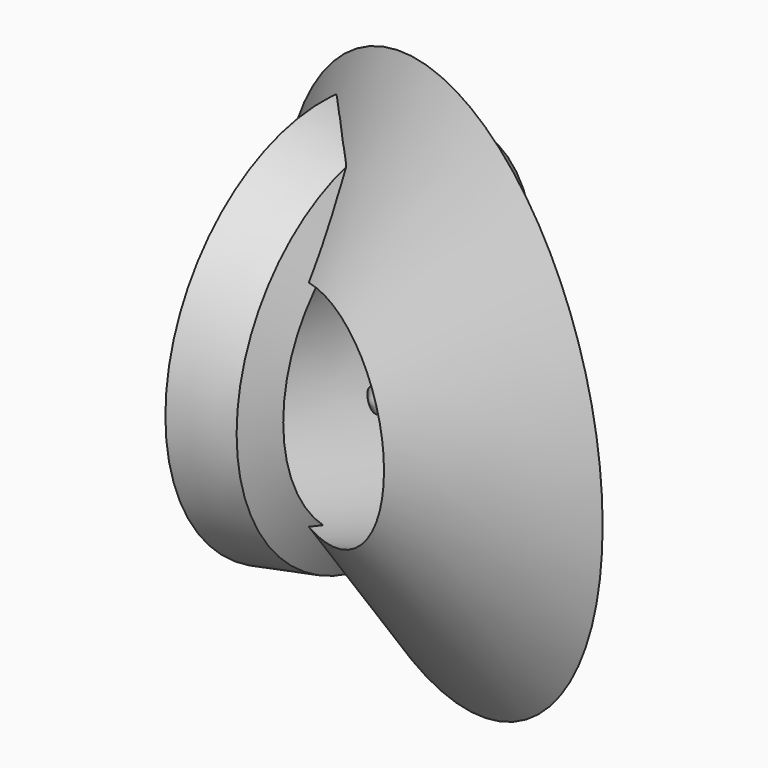
from build123d import *


# Not quite as in the source:
# - a feature of the source that left no trace in its solid (it failed there, or was rolled back) is left out


with BuildPart() as f2:
    # F0 (on Top) → F2 (revolve)
    with BuildSketch(Plane.XY):
        Polygon((41.6941601038, -6.1108729366), (29.3448964108, -6.1108729366), (17.3691271637, -21.2170399226), (36.609770419, -17.7606732331), align=None)
    revolve(axis=Axis((21.6941601038, 39.7148840129, 0), (1, 0, 0)))


with BuildPart() as f3:
    # F0 (on Top) → F3 (revolve)
    with BuildSketch(Plane.XY):
        Polygon((52.5221076777, 18.6990717526), (48.4309267247, 17.964136783), (51.0393636355, 15.3016783478), align=None)
    revolve(axis=Axis((41.6941601038, -6.1108729366, 0), (0.4, 0.916515139, 0)))


with BuildPart() as f3b:
    # F0 (on Top) → F3, piece 2 (revolve)
    with BuildSketch(Plane.XY):
        Polygon((107.4856412209, 28.5726567443), (76.4238416599, -10.6085199613), (135.4785561562, 0), align=None)
    revolve(axis=Axis((41.6941601038, -6.1108729366, 0), (0.4, 0.916515139, 0)))


solid = Compound([f2.part, f3.part, f3b.part])
